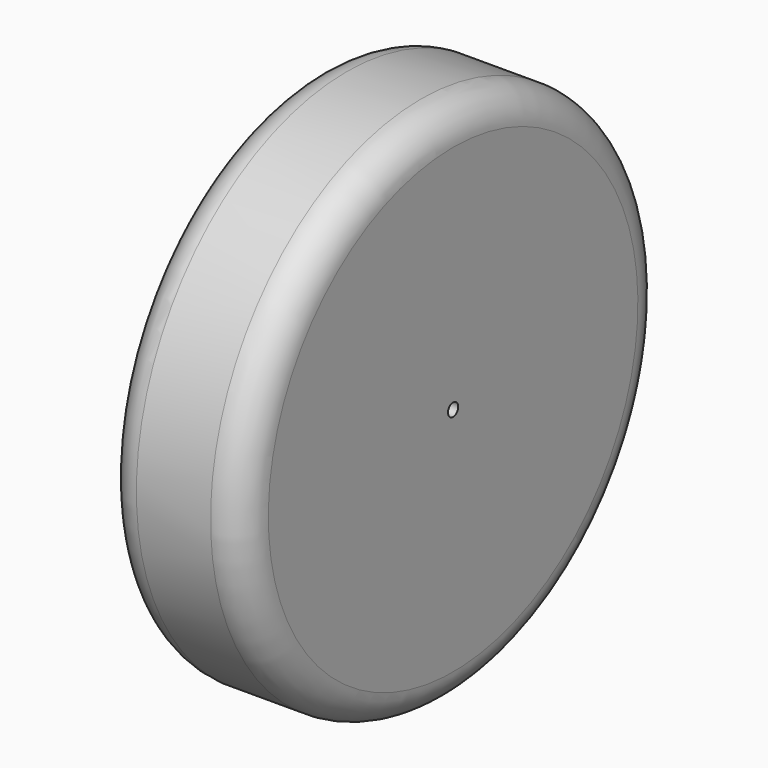
from build123d import *

# Parameters (mm, degrees)
F2_R = 5


# Not quite as in the source:
# - a feature names something its author has since deleted; it is built from what else it names


with BuildPart() as f1:
    # F0 (on Front) → F1 (revolve)
    with BuildSketch(Plane.XZ):
        Polygon((0, 5.4068532586), (-11.4892933807, 5.4068532586), (-11.4892933807, 1), (21.5621040944, 1), (21.5621040944, 41), (0, 41), align=None)
    revolve(axis=Axis((1.7312624663, 0, 0), (1, 0, 0)))

    # F2
    f2_edges = [f1.edges().sort_by_distance(p)[0] for p in [
        (21.562104, 0, -41),
        (0, 0, -41),
    ]]
    fillet(f2_edges, radius=F2_R)


solid = f1.part
